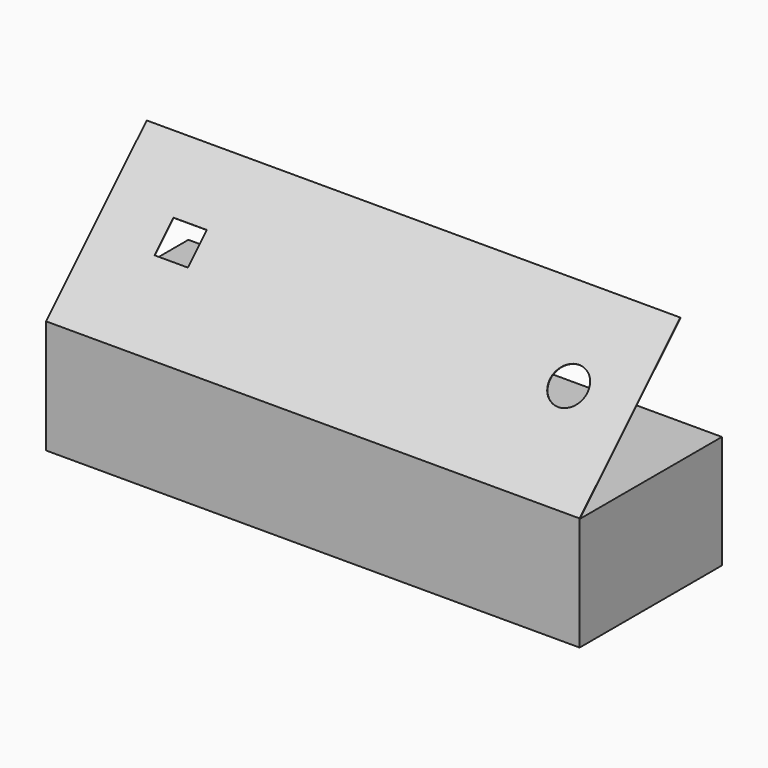
from build123d import *

# Parameters (mm, degrees)
F1_DEPTH = 209.55
F2_W     = 26.19375
F2_H     = 26.19375
F3_DEPTH = 0.4064


# Not quite as in the source:
# - the dataset's text gives a spline's control points without its knots; the knots are read off the source's solid


with BuildPart() as f1:
    # F0 (on Right) → F1 (new body, symmetric)
    with BuildSketch(Plane.YZ):
        Polygon((-139.7, 0), (0, 0), (0, 88.9), (-139.2936, 88.9), (-139.2936, 89.154), (-40.6298144724, 187.8177855276), (-40.9171826682, 188.1051537235), (-139.7, 89.3223363917), align=None)
    extrude(amount=F1_DEPTH, both=True)

    # F2 (on face) → F3 (cut, through all)
    with BuildSketch(Plane(origin=(0, -114.5111681959, 114.5111681959), x_dir=(1, 0, 0), z_dir=(0, -0.7071067812, 0.7071067812))):
        with Locations((-146.5093133926, 39.7379171954)):
            Rectangle(F2_W, F2_H)
        with BuildLine():
            add(Edge.make_bspline(
                [(168.6742066074, 50.1214371954), (165.9556700074, 52.8397705954), (162.1350528074, 54.4222921954), (158.2906866074, 54.4222921954)],
                knots=[7, 7, 7, 7, 8, 8, 8, 8], degree=3))
            add(Edge.make_bspline(
                [(158.2906866074, 54.4222921954), (154.4462950074, 54.4222921954), (150.6256778074, 52.8397705954), (147.9074968074, 50.1214371954)],
                knots=[0, 0, 0, 0, 1, 1, 1, 1], degree=3))
            add(Edge.make_bspline(
                [(147.9074968074, 50.1214371954), (145.1889856074, 47.4029005954), (143.6063116074, 43.5822833954), (143.6063116074, 39.7379171954), (143.6063116074, 35.8935255954), (145.1889856074, 32.0729083954), (147.9074968074, 29.3543971954)],
                knots=[1, 1, 1, 1, 2, 2, 2, 3, 3, 3, 3], degree=3))
            add(Edge.make_bspline(
                [(147.9074968074, 29.3543971954), (150.6256778074, 26.6360383954), (154.4462950074, 25.0535421954), (158.2906866074, 25.0535421954), (162.1350528074, 25.0535421954), (165.9556700074, 26.6360383954), (168.6742066074, 29.3543971954)],
                knots=[3, 3, 3, 3, 4, 4, 4, 5, 5, 5, 5], degree=3))
            add(Edge.make_bspline(
                [(168.6742066074, 29.3543971954), (171.3927178074, 32.0729083954), (172.9750616074, 35.8935255954), (172.9750616074, 39.7379171954), (172.9750616074, 43.5822833954), (171.3927178074, 47.4029005954), (168.6742066074, 50.1214371954)],
                knots=[5, 5, 5, 5, 6, 6, 6, 7, 7, 7, 7], degree=3))
        make_face()
    extrude(amount=-F3_DEPTH, mode=Mode.SUBTRACT)


solid = f1.part
